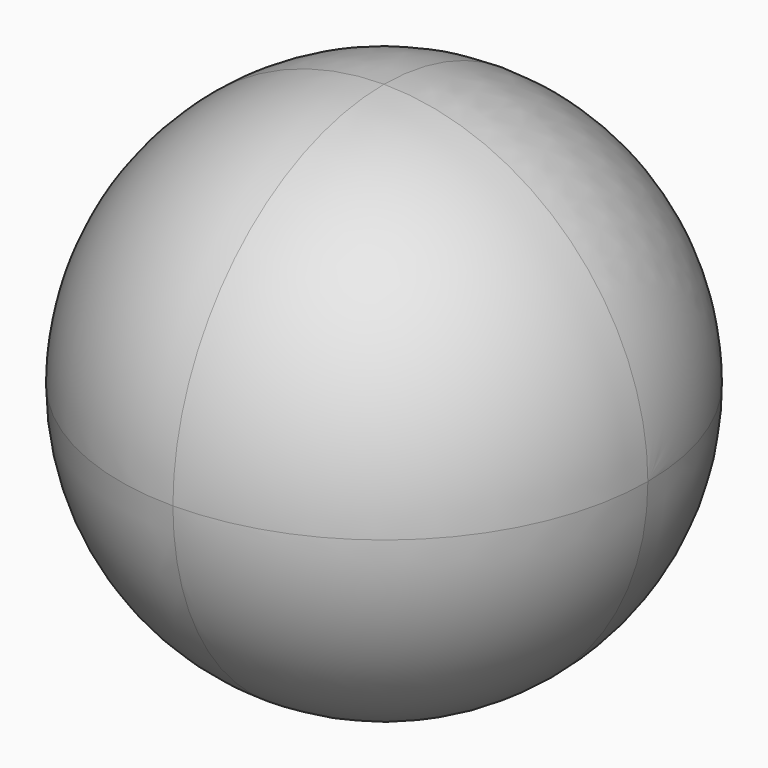
from build123d import *

# Parameters (mm, degrees)
F0_W        = 200
F0_H        = 200
F1_DEPTH    = 200
F2_R        = 99.99999
F3_T1_DEPTH = 200
F3_T4_ANGLE = 90
F3_T6_ANGLE = 90


# Not quite as in the source:
# - a fillet or chamfer that OpenCascade refuses, or shapes differently, is made with other operations: its cross-section is extruded or revolved along the edge and cut away or added
# - a fillet or chamfer is up to 0.001 mm smaller than in the source, because OpenCascade refuses the exact size


with BuildPart() as f1:
    # F0 (on Front) → F1 (new body)
    with BuildSketch(Plane.XZ):
        Rectangle(F0_W, F0_H)
    extrude(amount=F1_DEPTH)

    # F2 (radius 100 in the source; OpenCascade refuses exactly that, so slightly less here)
    f2_edges = [f1.edges().sort_by_distance(p)[0] for p in [
        (100, -100, -100),
        (100, -100, 100),
        (100, 0, 0),
        (100, -200, 0),
        (0, -200, 100),
        (-100, -200, 0),
        (0, -200, -100),
        (-100, -100, -100),
        (0, 0, -100),
        (-100, -100, 100),
        (-100, 0, 0),
    ]]
    fillet(f2_edges, radius=F2_R)

    # F3: fillet of radius 100 on 1 edges, made by hand

    # F3_s2 → F3_t1 (cut)
    with BuildSketch(Plane.YZ.offset(-100)):
        with BuildLine():
            ThreePointArc((0, 0), (-29.2893218813, 70.7106781187), (-100, 100))
            Line((-100, 100), (0, 100))
            Line((0, 100), (0, 0))
        make_face()
    extrude(amount=F3_T1_DEPTH, mode=Mode.SUBTRACT)

    # F3_s3 → F3_t4 (revolve, cut)
    with BuildSketch(Plane.XY):
        with BuildLine():
            ThreePointArc((100, -99.99999), (70.7106810476, -29.2893189524), (1e-05, 0))
            Line((1e-05, 0), (100, 0))
            Line((100, 0), (100, -99.99999))
        make_face()
    revolve(axis=Axis((100, -100, 0), (1, 0, 0)), revolution_arc=F3_T4_ANGLE, mode=Mode.SUBTRACT)

    # F3_s5 → F3_t6 (revolve, cut)
    with BuildSketch(Plane.XZ.offset(100)):
        with BuildLine():
            ThreePointArc((-100, 1e-05), (-70.7106810476, 70.7106810476), (-1e-05, 100))
            Line((-1e-05, 100), (-100, 100))
            Line((-100, 100), (-100, 1e-05))
        make_face()
    revolve(axis=Axis((-100, -100, 0), (-1, 0, 0)), revolution_arc=F3_T6_ANGLE, mode=Mode.SUBTRACT)


solid = f1.part
